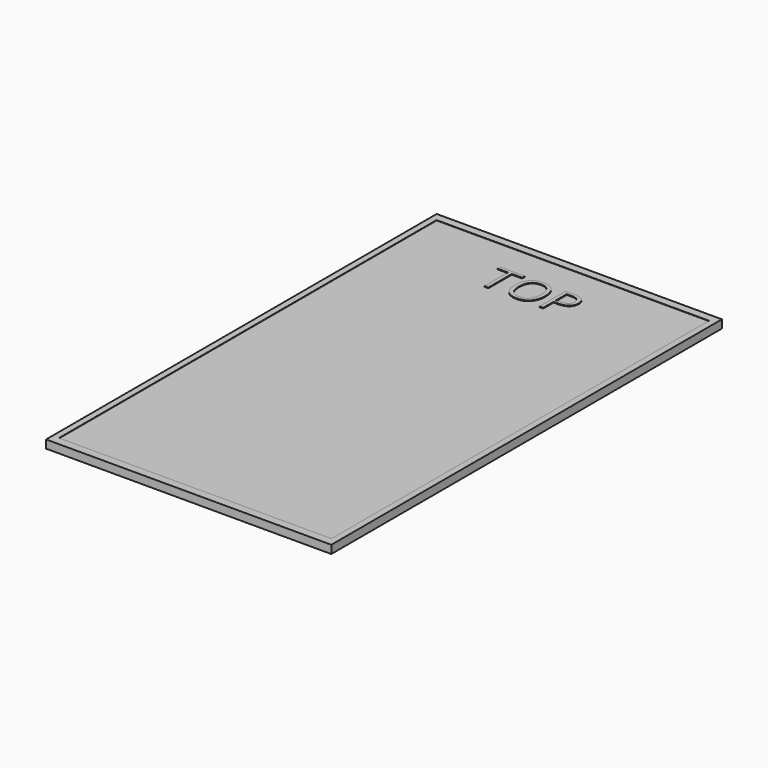
from build123d import *

# Parameters (mm, degrees)
F0_W         = 209.55
F0_H         = 358.775
F1_DEPTH     = 6
F2_W         = 200.15
F2_H         = 346.775
F3_DEPTH     = 0.25
F4_TEXT_SIZE = 33.7089308434
F5_DEPTH     = 0.5
F7_DEPTH     = 1


# Not quite as in the source:
# - Text() gives the source's letters only with a copy of the font that has no kerning and outlines rounded to 1/6400 em; it was checked with that copy


with BuildPart() as f1:
    # F0 (on Top) → F1 (new body)
    with BuildSketch(Plane.XY):
        Rectangle(F0_W, F0_H)
    extrude(amount=F1_DEPTH)

    # F2 (on face) → F3 (cut)
    with BuildSketch(Plane.XY.offset(6)):
        Rectangle(F2_W, F2_H)
    extrude(amount=-F3_DEPTH, mode=Mode.SUBTRACT)

    # F4 (on face) → F5 (join)
    with BuildSketch(Plane.XY.offset(5.75)):
        with Locations((-34.9557213485, 126.1614710093)):
            Text('TOP', F4_TEXT_SIZE, font='Open Sans', text_align=(TextAlign.LEFT, TextAlign.BOTTOM))
    extrude(amount=F5_DEPTH)

    # F6 (on face) → F7 (join)
    with BuildSketch(Plane(origin=(0, 0, 0), x_dir=(1, 0, 0), z_dir=(0, 0, -1))):
        Polygon((-72.6724788547, 159.8882228136), (-72.6724788547, -7.9353442416), (-57.2748966515, -7.9353442416), (-57.2748966515, 29.0618762374), (-61.8732124567, 29.0618762374), (-61.8732124567, 65.8483803272), (-57.2748966515, 65.8483803272), (-57.2748966515, 159.8882228136), align=None)
        Polygon((-99.564820528, 159.8882228136), (-99.564820528, -161.2766832113), (-72.6724788547, -161.2766832113), (-72.6724788547, -7.9353442416), (-72.6724788547, 159.8882228136), align=None)
    extrude(amount=F7_DEPTH)


solid = f1.part
